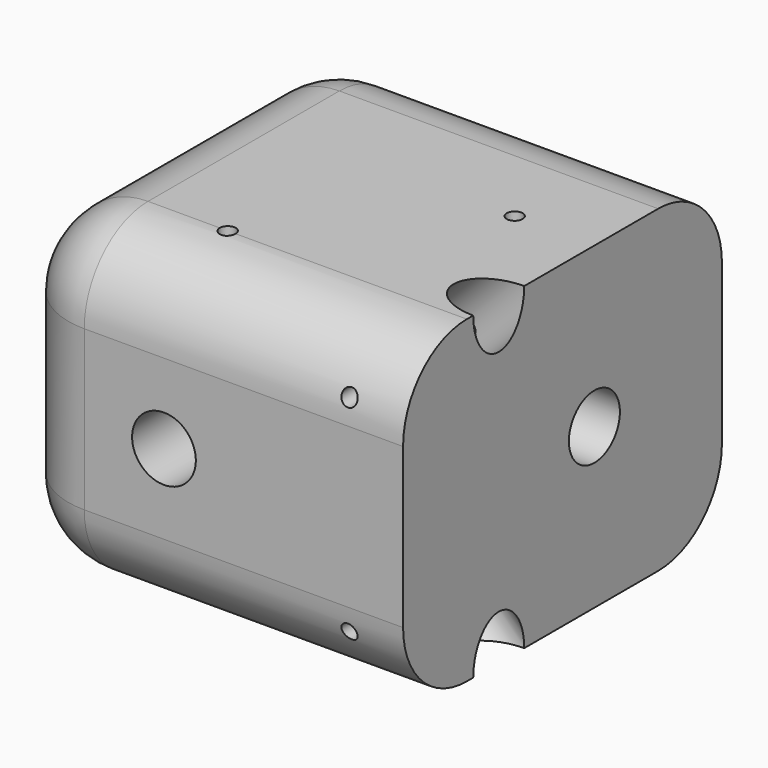
from build123d import *

# Parameters (mm, degrees)
F0_W          = 30
F0_H          = 30
F1_DEPTH      = 20
F2_R          = 2
F3_DEPTH      = 15
F4_R          = 2
F4_R_2        = 0.5
F5_DEPTH      = 15
F7_R          = 2
F8_DEPTH      = 15
F10_R         = 2
F11_DEPTH     = 15
F12_R         = 0.5
F13_DEPTH     = 20.0010001
F14_T1_DEPTH  = 10
F14_T3_DEPTH  = 32.5
F14_T5_DEPTH  = 15
F14_S9_W      = 5
F14_S9_H      = 5
F14_T10_DEPTH = 5
F14_S15_W     = 5
F14_S15_H     = 5
F14_T16_DEPTH = 5
F14_S21_W     = 5
F14_S21_H     = 5
F14_T22_DEPTH = 5
F14_S27_W     = 5
F14_S27_H     = 5
F14_T28_DEPTH = 5


# Not quite as in the source:
# - a fillet or chamfer that OpenCascade refuses, or shapes differently, is made with other operations: its cross-section is extruded or revolved along the edge and cut away or added


with BuildPart() as f1:
    # F0 (on Top) → F1 (new body)
    with BuildSketch(Plane.XY):
        Rectangle(F0_W, F0_H)
    extrude(amount=F1_DEPTH)

    # F2 (on face) → F3 (cut)
    with BuildSketch(Plane.YZ.offset(15)):
        with Locations((0, 10)):
            Circle(F2_R)
    extrude(amount=-F3_DEPTH, mode=Mode.SUBTRACT)

    # F4 (on face) → F5 (cut)
    with BuildSketch(Plane.XZ.offset(15)):
        with Locations((0, 10)):
            Circle(F4_R)
        with Locations((11.4644660941, 16.4644660941)):
            Circle(F4_R_2)
        with Locations((11.4644660941, 3.5355339059)):
            Circle(F4_R_2)
    extrude(amount=-F5_DEPTH, mode=Mode.SUBTRACT)

    # F7 (on face) → F8 (cut)
    with BuildSketch(Plane(origin=(17.5, 0, 17.5), x_dir=(0, 1, 0), z_dir=(0.7071067812, 0, 0.7071067812))):
        with Locations((-7.5, 3.5355339059)):
            Circle(F7_R)
    extrude(amount=-F8_DEPTH, mode=Mode.SUBTRACT)

    # F10 (on face) → F11 (cut)
    with BuildSketch(Plane(origin=(7.5, 0, -7.5), x_dir=(0.7071067812, 0, 0.7071067812), z_dir=(0.7071067812, 0, -0.7071067812))):
        with Locations((10.6066017178, 7.5)):
            Circle(F10_R)
    extrude(amount=-F11_DEPTH, mode=Mode.SUBTRACT)

    # F12 (on face) → F13 (cut, through all)
    with BuildSketch(Plane.XY.offset(20)):
        Polygon((-60, -15), (-10, -15), (-10, 10), (15, 10), (15, 50), (-60, 50), align=None)
        with Locations((10, 0)):
            Circle(F12_R)
        with Locations((0, -10)):
            Circle(F12_R)
    extrude(amount=-F13_DEPTH, mode=Mode.SUBTRACT)

    # F14: fillet of radius 5 on 8 edges, made by hand

    # F14_s2 → F14_t1 (cut)
    with BuildSketch(Plane.XY.offset(5)):
        with BuildLine():
            ThreePointArc((-5, -15), (-8.5355339059, -13.5355339059), (-10, -10))
            Line((-10, -10), (-10, -15))
            Line((-10, -15), (-5, -15))
        make_face()
        with BuildLine():
            ThreePointArc((-5, 10), (-8.5355339059, 8.5355339059), (-10, 5))
            Line((-10, 5), (-10, 10))
            Line((-10, 10), (-5, 10))
        make_face()
    extrude(amount=F14_T1_DEPTH, mode=Mode.SUBTRACT)

    # F14_s4 → F14_t3 (cut)
    with BuildSketch(Plane.YZ.offset(-5)):
        with BuildLine():
            ThreePointArc((-10, 20), (-13.5355339059, 18.5355339059), (-15, 15))
            Line((-15, 15), (-15, 20))
            Line((-15, 20), (-10, 20))
        make_face()
        with BuildLine():
            ThreePointArc((10, 15), (8.5355339059, 18.5355339059), (5, 20))
            Line((5, 20), (10, 20))
            Line((10, 20), (10, 15))
        make_face()
        with BuildLine():
            ThreePointArc((5, 0), (8.5355339059, 1.4644660941), (10, 5))
            Line((10, 5), (10, 0))
            Line((10, 0), (5, 0))
        make_face()
        with BuildLine():
            ThreePointArc((-10, 0), (-13.5355339059, 1.4644660941), (-15, 5))
            Line((-15, 5), (-15, 0))
            Line((-15, 0), (-10, 0))
        make_face()
    extrude(amount=F14_T3_DEPTH, mode=Mode.SUBTRACT)

    # F14_s6 → F14_t5 (cut)
    with BuildSketch(Plane.XZ.offset(-5)):
        with BuildLine():
            ThreePointArc((-5, 20), (-8.5355339059, 18.5355339059), (-10, 15))
            Line((-10, 15), (-10, 20))
            Line((-10, 20), (-5, 20))
        make_face()
        with BuildLine():
            ThreePointArc((-5, 0), (-8.5355339059, 1.4644660941), (-10, 5))
            Line((-10, 5), (-10, 0))
            Line((-10, 0), (-5, 0))
        make_face()
    extrude(amount=F14_T5_DEPTH, mode=Mode.SUBTRACT)


with BuildPart() as f14_tool8:
    # F14_s9 → F14_t10 (new body)
    with BuildSketch(Plane.YZ.offset(-5)):
        with Locations((-12.5, 17.5)):
            Rectangle(F14_S9_W, F14_S9_H)
    extrude(amount=-F14_T10_DEPTH)

    # F14_s11 → F14_t12 (revolve, cut)
    with BuildSketch(Plane(origin=(-5, -10, 15), x_dir=(0, 0.7071067812, -0.7071067812), z_dir=(0, 0.7071067812, 0.7071067812))):
        with BuildLine():
            ThreePointArc((0, -5), (5, 0), (0, 5))
            Line((0, 5), (0, -5))
        make_face()
    revolve(axis=Axis((-5, -10, 15), (-1, 0, 0)), mode=Mode.SUBTRACT)


with BuildPart() as f1_1:
    add(f1.part)

    # F14_t7: cut F14_tool8
    add(f14_tool8.part, mode=Mode.SUBTRACT)


with BuildPart() as f14_tool14:
    # F14_s15 → F14_t16 (new body)
    with BuildSketch(Plane.YZ.offset(-5)):
        with Locations((-12.5, 2.5)):
            Rectangle(F14_S15_W, F14_S15_H)
    extrude(amount=-F14_T16_DEPTH)

    # F14_s17 → F14_t18 (revolve, cut)
    with BuildSketch(Plane(origin=(-5, -10, 5), x_dir=(0, 0.7071067812, 0.7071067812), z_dir=(0, -0.7071067812, 0.7071067812))):
        with BuildLine():
            ThreePointArc((0, -5), (5, 0), (0, 5))
            Line((0, 5), (0, -5))
        make_face()
    revolve(axis=Axis((-5, -10, 5), (-1, 0, 0)), mode=Mode.SUBTRACT)


with BuildPart() as f1_2:
    add(f1_1.part)

    # F14_t13: cut F14_tool14
    add(f14_tool14.part, mode=Mode.SUBTRACT)


with BuildPart() as f14_tool20:
    # F14_s21 → F14_t22 (new body)
    with BuildSketch(Plane.YZ.offset(-5)):
        with Locations((7.5, 17.5)):
            Rectangle(F14_S21_W, F14_S21_H)
    extrude(amount=-F14_T22_DEPTH)

    # F14_s23 → F14_t24 (revolve, cut)
    with BuildSketch(Plane(origin=(-5, 5, 15), x_dir=(0, -0.7071067812, -0.7071067812), z_dir=(0, 0.7071067812, -0.7071067812))):
        with BuildLine():
            ThreePointArc((0, -5), (5, 0), (0, 5))
            Line((0, 5), (0, -5))
        make_face()
    revolve(axis=Axis((-5, 5, 15), (-1, 0, 0)), mode=Mode.SUBTRACT)


with BuildPart() as f1_3:
    add(f1_2.part)

    # F14_t19: cut F14_tool20
    add(f14_tool20.part, mode=Mode.SUBTRACT)


with BuildPart() as f14_tool26:
    # F14_s27 → F14_t28 (new body)
    with BuildSketch(Plane.YZ.offset(-5)):
        with Locations((7.5, 2.5)):
            Rectangle(F14_S27_W, F14_S27_H)
    extrude(amount=-F14_T28_DEPTH)

    # F14_s29 → F14_t30 (revolve, cut)
    with BuildSketch(Plane(origin=(-5, 5, 5), x_dir=(0, -0.7071067812, 0.7071067812), z_dir=(0, -0.7071067812, -0.7071067812))):
        with BuildLine():
            ThreePointArc((0, -5), (5, 0), (0, 5))
            Line((0, 5), (0, -5))
        make_face()
    revolve(axis=Axis((-5, 5, 5), (-1, 0, 0)), mode=Mode.SUBTRACT)


with BuildPart() as f1_4:
    add(f1_3.part)

    # F14_t25: cut F14_tool26
    add(f14_tool26.part, mode=Mode.SUBTRACT)


solid = f1_4.part
